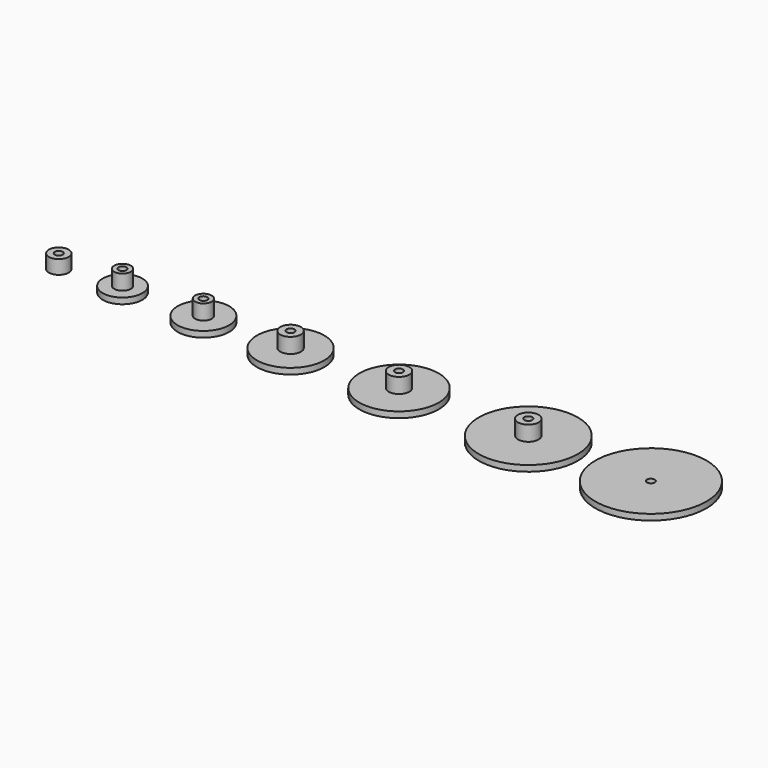
from build123d import *

# Parameters (mm, degrees)
F0_R      = 8.5
F0_R_2    = 1
F1_DEPTH  = 1.5
F2_R      = 2.6
F2_R_2    = 1
F3_DEPTH  = 3.8
F4_R      = 10
F4_R_2    = 1
F5_DEPTH  = 1.5
F4_R_3    = 12.5
F4_R_4    = 6.5
F4_R_5    = 5
F4_R_6    = 2.5
F6_R      = 2.6
F6_R_2    = 1
F7_DEPTH  = 3.8
F8_R      = 2.6
F8_R_2    = 1
F9_DEPTH  = 3.8
F10_R     = 2.1
F10_R_2   = 1
F11_DEPTH = 3.8
F12_R     = 2.1
F12_R_2   = 1
F13_DEPTH = 3.8
F14_DEPTH = 2
F15_R     = 14
F15_R_2   = 1
F16_DEPTH = 1.5


# Not quite as in the source:
# - a feature names something its author has since deleted; it is built from what else it names


with BuildPart() as f1:
    # F0 (on Top) → F1 (new body)
    with BuildSketch(Plane.XY):
        Circle(F0_R)
        Circle(F0_R_2, mode=Mode.SUBTRACT)
    extrude(amount=F1_DEPTH)

    # F2 (on face) → F3 (join)
    with BuildSketch(Plane.XY.offset(1.5)):
        Circle(F2_R)
        Circle(F2_R_2, mode=Mode.SUBTRACT)
    extrude(amount=F3_DEPTH)


with BuildPart() as f5:
    # F4 (on Top) → F5 (new body)
    with BuildSketch(Plane.XY):
        with Locations((27.3370184205, 0)):
            Circle(F4_R)
        with Locations((27.3370184205, 0)):
            Circle(F4_R_2, mode=Mode.SUBTRACT)
    extrude(amount=F5_DEPTH)

    # F6 (on face) → F7 (join)
    with BuildSketch(Plane.XY.offset(1.5)):
        with Locations((27.3370184205, 0)):
            Circle(F6_R)
        with Locations((27.3370184205, 0)):
            Circle(F6_R_2, mode=Mode.SUBTRACT)
    extrude(amount=F7_DEPTH)


with BuildPart() as f5b:
    # F4 (on Top) → F5, piece 2 (new body)
    with BuildSketch(Plane.XY):
        with Locations((59.9259639982, 0)):
            Circle(F4_R_3)
        with Locations((59.9259639982, 0)):
            Circle(F4_R_2, mode=Mode.SUBTRACT)
    extrude(amount=F5_DEPTH)

    # F8 (on face) → F9 (join)
    with BuildSketch(Plane.XY.offset(1.5)):
        with Locations((59.9259639982, 0)):
            Circle(F8_R)
        with Locations((59.9259639982, 0)):
            Circle(F8_R_2, mode=Mode.SUBTRACT)
    extrude(amount=F9_DEPTH)


with BuildPart() as f5c:
    # F4 (on Top) → F5, piece 3 (new body)
    with BuildSketch(Plane.XY):
        with Locations((-21.9778250903, 0)):
            Circle(F4_R_4)
        with Locations((-21.9778250903, 0)):
            Circle(F4_R_2, mode=Mode.SUBTRACT)
    extrude(amount=F5_DEPTH)

    # F10 (on face) → F11 (join)
    with BuildSketch(Plane.XY.offset(1.5)):
        with Locations((-21.9778250903, 0)):
            Circle(F10_R)
        with Locations((-21.9778250903, 0)):
            Circle(F10_R_2, mode=Mode.SUBTRACT)
    extrude(amount=F11_DEPTH)


with BuildPart() as f5d:
    # F4 (on Top) → F5, piece 4 (new body)
    with BuildSketch(Plane.XY):
        with Locations((-42.3665866256, 0)):
            Circle(F4_R_5)
        with Locations((-42.3665866256, 0)):
            Circle(F4_R_2, mode=Mode.SUBTRACT)
    extrude(amount=F5_DEPTH)

    # F12 (on face) → F13 (join)
    with BuildSketch(Plane.XY.offset(1.5)):
        with Locations((-42.3665866256, 0)):
            Circle(F12_R)
        with Locations((-42.3665866256, 0)):
            Circle(F12_R_2, mode=Mode.SUBTRACT)
    extrude(amount=F13_DEPTH)


with BuildPart() as f5e:
    # F4 (on Top) → F5, piece 5 (new body)
    with BuildSketch(Plane.XY):
        with Locations((-58.4356933832, 0)):
            Circle(F4_R_6)
        with Locations((-58.4356933832, 0)):
            Circle(F4_R_2, mode=Mode.SUBTRACT)
    extrude(amount=F5_DEPTH)

    # F14 (add): a face of the model
    f14_faces = [f5e.faces().sort_by_distance(p)[0] for p in [
        (-60.8649827051, 0, 1.5),
    ]]
    extrude(f14_faces, amount=F14_DEPTH)


with BuildPart() as f16:
    # F15 (on Top) → F16 (new body)
    with BuildSketch(Plane.XY):
        with Locations((90.8367805009, 0)):
            Circle(F15_R)
        with Locations((90.8367805009, 0)):
            Circle(F15_R_2, mode=Mode.SUBTRACT)
    extrude(amount=F16_DEPTH)


solid = Compound([f1.part, f5.part, f5b.part, f5c.part, f5d.part, f5e.part, f16.part])
